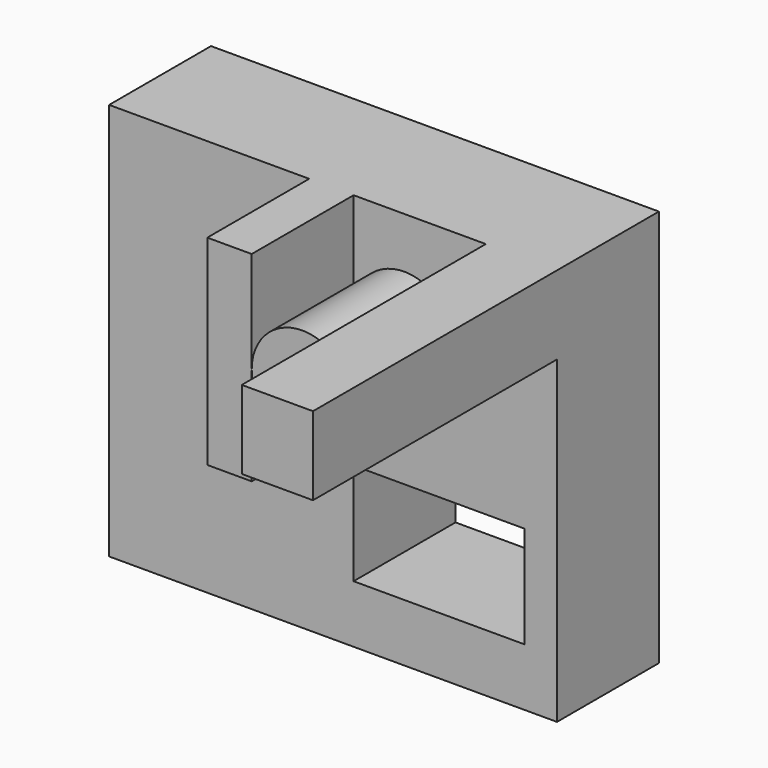
from build123d import *

# Parameters (mm, degrees)
F0_W     = 89.3156863749
F0_H     = 79.2764052749
F1_DEPTH = 25.4
F2_W     = 14.1974128783
F2_H     = 15.6361199915
F3_DEPTH = 60.8264654875
F4_W     = 34.0766403824
F4_H     = 20.3113891184
F5_DEPTH = 25.4
F6_R     = 10.1085053757
F7_DEPTH = 25.4
F9_DEPTH = 25.4


with BuildPart() as f1:
    # F0 (on Front) → F1 (new body)
    with BuildSketch(Plane.XZ):
        with Locations((4.7579761595, 0.2727396786)):
            Rectangle(F0_W, F0_H)
    extrude(amount=F1_DEPTH)

    # F2 (on face) → F3 (join)
    with BuildSketch(Plane.XZ.offset(25.4)):
        with Locations((42.3171129078, 32.0928823203)):
            Rectangle(F2_W, F2_H)
    extrude(amount=F3_DEPTH)

    # F4 (on face) → F5 (cut)
    with BuildSketch(Plane.XZ.offset(25.4)):
        with Locations((25.8919894695, -17.7010148764)):
            Rectangle(F4_W, F4_H)
    extrude(amount=-F5_DEPTH, mode=Mode.SUBTRACT)

    # F6 (on face) → F7 (cut)
    with BuildSketch(Plane(origin=(0, 0, 0), x_dir=(-1, 0, 0), z_dir=(0, 1, 0))):
        with Locations((-18.962174654, 19.6714401245)):
            Circle(F6_R)
    extrude(amount=-F7_DEPTH, mode=Mode.SUBTRACT)

    # F8 (on face) → F9 (join)
    with BuildSketch(Plane.XZ.offset(25.4)):
        Polygon((8.8536692783, 19.6714401245), (8.8536692783, 39.9109423161), (0, 39.9109423161), (0, 0), (8.8536692783, 0), align=None)
    extrude(amount=F9_DEPTH)


with BuildPart() as f9:
    # F8 (on face) → F9, piece 2 (new body)
    with BuildSketch(Plane.XZ.offset(25.4)):
        with BuildLine():
            ThreePointArc((29.0706800297, 19.6714401245), (18.962174654, 29.7799455002), (8.8536692783, 19.6714401245))
            ThreePointArc((8.8536692783, 19.6714401245), (18.962174654, 9.5629347488), (29.0706800297, 19.6714401245))
        make_face()
    extrude(amount=F9_DEPTH)


solid = Compound([f1.part, f9.part])
